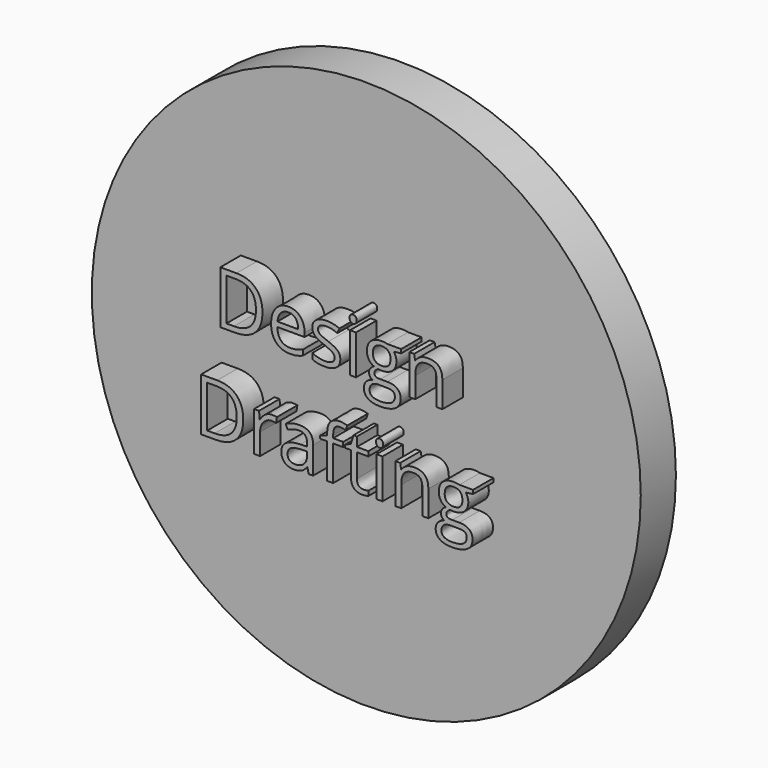
from build123d import *

# Parameters (mm, degrees)
F1_TEXT_SIZE = 20.203027331
F2_DEPTH     = 7
F0_R         = 75
F3_DEPTH     = 12


# Not quite as in the source:
# - Text() gives the source's letters only with a copy of the font that has no kerning and outlines rounded to 1/6400 em; it was checked with that copy


with BuildPart() as f2:
    # F1 (on Front) → F2 (new body)
    with BuildSketch(Plane.XZ):
        with Locations((-36.2739030246, 7.7830421578)):
            Text('Design', F1_TEXT_SIZE, font='Open Sans', text_align=(TextAlign.LEFT, TextAlign.BOTTOM))
        with Locations((-41.5235334076, -19.6930750123)):
            Text('Drafting', F1_TEXT_SIZE, font='Open Sans', text_align=(TextAlign.LEFT, TextAlign.BOTTOM))
    extrude(amount=F2_DEPTH)

    # F0 (on Front) → F3 (join)
    with BuildSketch(Plane.XZ):
        Circle(F0_R)
    extrude(amount=-F3_DEPTH)


solid = f2.part
